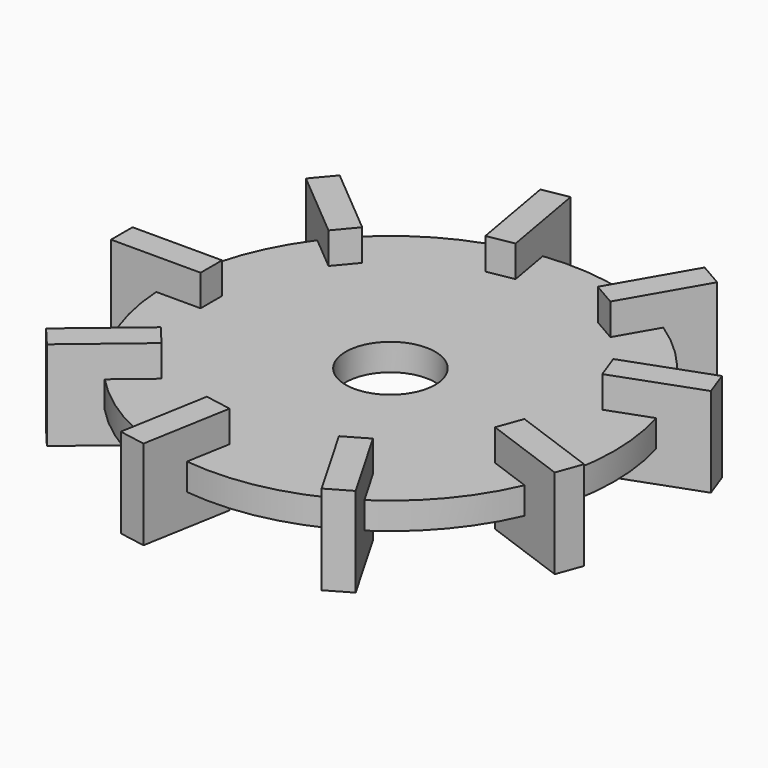
from build123d import *

# Parameters (mm, degrees)
F0_R            = 63.5
F0_R_2          = 12.7
F2_DEPTH        = 3.81
F1_W            = 25.4
F1_H            = 3.81
F3_DEPTH        = 12.7
F3_COPIES_COUNT = 9


# Not quite as in the source:
# - a pattern or mirror of a feature is missing from the dataset's text; its kind, count and spacing are read off the source's solid


with BuildPart() as f2:
    # F0 (on Top) → F2 (new body, symmetric)
    with BuildSketch(Plane.XY):
        Circle(F0_R)
        Circle(F0_R_2, mode=Mode.SUBTRACT)
    extrude(amount=F2_DEPTH, both=True)

    # F1 (on Top) → F3 (join, symmetric)
    with BuildSketch(Plane.XY):
        with Locations((-63.5, 1.905)):
            Rectangle(F1_W, F1_H)
        with Locations((-63.5, -1.905)):
            Rectangle(F1_W, F1_H)
    f3 = extrude(amount=F3_DEPTH, both=True)

    # F3_copies: F3 ×9 about axis
    f3_copies_axis = Axis((0, 0, 0), (0, 0, 1))
    for i in range(1, F3_COPIES_COUNT):
        add(f3.rotate(f3_copies_axis, i * 360 / F3_COPIES_COUNT))


solid = f2.part
